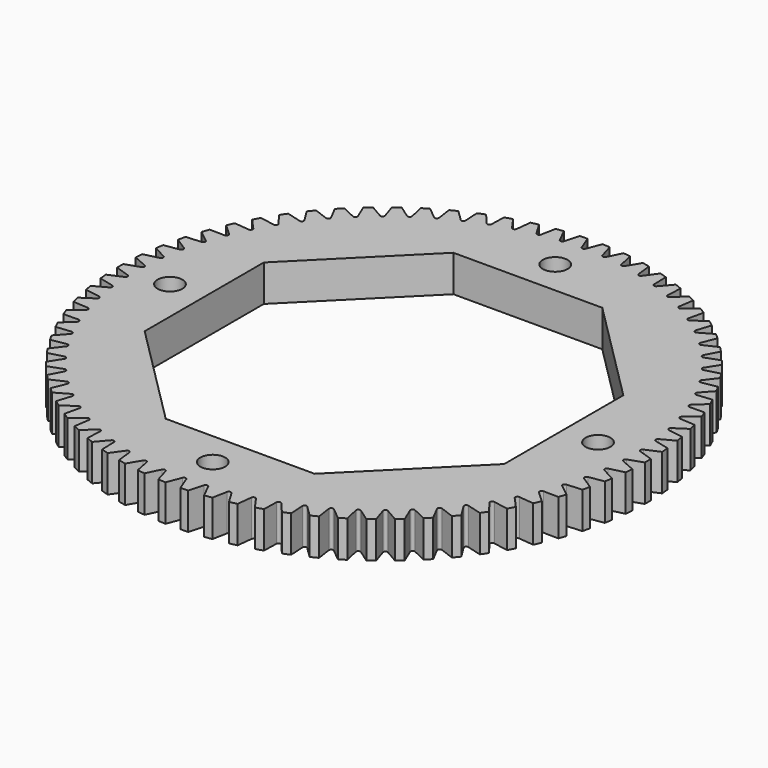
from build123d import *

# Parameters (mm, degrees)
F0_R            = 36.6966028895
F0_R_2          = 1.7272
F1_DEPTH        = 5.08
F3_DEPTH        = 5.08
F3_COPIES_COUNT = 74


# Not quite as in the source:
# - a pattern or mirror of a feature is missing from the dataset's text; its kind, count and spacing are read off the source's solid


with BuildPart() as f1:
    # F0 (on Top) → F1 (new body)
    with BuildSketch(Plane.XY):
        Circle(F0_R)
        with Locations((0, -29.7625)):
            Circle(F0_R_2, mode=Mode.SUBTRACT)
        with Locations((-29.7625, 0)):
            Circle(F0_R_2, mode=Mode.SUBTRACT)
        Polygon((25, -10.3553390593), (10.3553390593, -25), (-10.3553390593, -25), (-25, -10.3553390593), (-25, 10.3553390593), (-10.3553390593, 25), (10.3553390593, 25), (25, 10.3553390593), align=None, mode=Mode.SUBTRACT)
        with Locations((29.7625, 0)):
            Circle(F0_R_2, mode=Mode.SUBTRACT)
        with Locations((0, 29.7625)):
            Circle(F0_R_2, mode=Mode.SUBTRACT)
    extrude(amount=F1_DEPTH)

    # F2 (on face) → F3 (cut, through all)
    with BuildSketch(Plane(origin=(0, 0, 0), x_dir=(1, 0, 0), z_dir=(0, 0, -1))):
        with BuildLine():
            Line((0.2776832038, 34.7226938161), (1.0318138612, 36.6820940485))
            ThreePointArc((1.0318138612, 36.6820940485), (0, 36.6966028895), (-1.0318138612, 36.6820940485))
            Line((-1.0318138612, 36.6820940485), (-0.2776832038, 34.7226938161))
            ThreePointArc((-0.2776832038, 34.7226938161), (0, 34.5320280359), (0.2776832038, 34.7226938161))
        make_face()
    f3 = extrude(amount=-F3_DEPTH, mode=Mode.SUBTRACT)

    # F3_copies: F3 ×74 about axis
    f3_copies_axis = Axis((0, 0, 0), (0, 0, 1))
    for i in range(1, F3_COPIES_COUNT):
        add(f3.rotate(f3_copies_axis, i * 360 / F3_COPIES_COUNT), mode=Mode.SUBTRACT)


solid = f1.part
